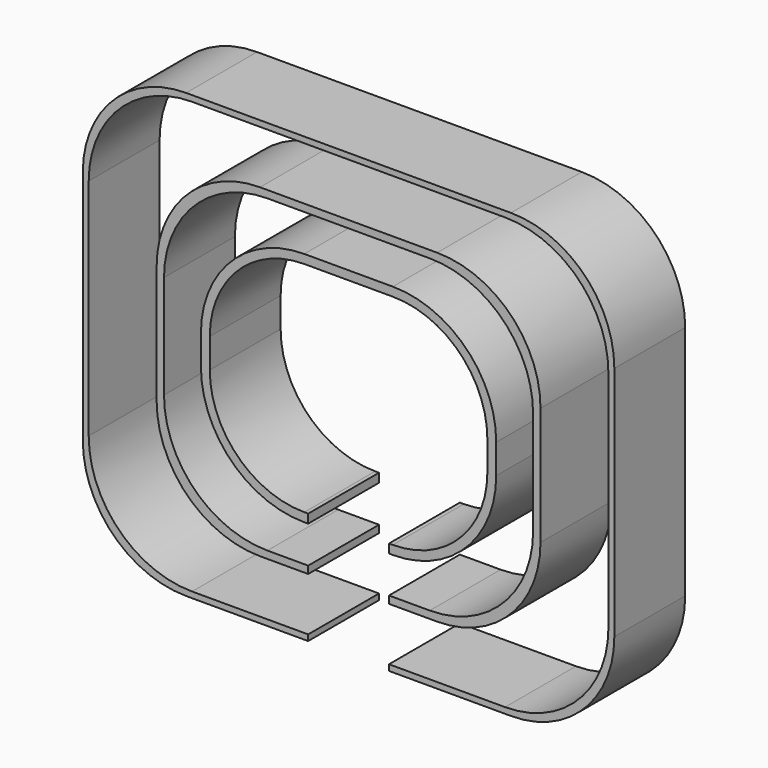
from build123d import *

# Parameters (mm, degrees)
F0_W      = 180
F0_H      = 150
F1_DEPTH  = 30
F2_T      = -2
F3_W      = 130
F3_H      = 110
F4_DEPTH  = 30
F5_T      = -2.5
F6_W      = 100
F6_H      = 80
F7_DEPTH  = 30
F8_R      = 35
F8_2_R    = 35
F8_3_R    = 35
F9_T      = -3
F10_W     = 27.3726535961
F10_H     = 91.242223978
F11_DEPTH = 30.001


with BuildPart() as f1:
    # F0 (on Front) → F1 (new body)
    with BuildSketch(Plane.XZ):
        Rectangle(F0_W, F0_H)
    extrude(amount=F1_DEPTH)

    # F2
    f2_openings = [f1.faces().sort_by_distance(p)[0] for p in [
        (0, -30, 0),
        (0, 0, 0),
    ]]
    offset(amount=F2_T, openings=f2_openings)

    # F8
    f8_edges = [f1.edges().sort_by_distance(p)[0] for p in [
        (-88, -15, 73),
        (-90, -15, 75),
        (90, -15, 75),
        (88, -15, 73),
        (88, -15, -73),
        (90, -15, -75),
        (-88, -15, -73),
        (-90, -15, -75),
    ]]
    fillet(f8_edges, radius=F8_R)


with BuildPart() as f4:
    # F3 (on face) → F4 (new body)
    with BuildSketch(Plane.XZ):
        Rectangle(F3_W, F3_H)
    extrude(amount=F4_DEPTH)

    # F5
    f5_openings = [f4.faces().sort_by_distance(p)[0] for p in [
        (0, -30, 0),
        (0, 0, 0),
    ]]
    offset(amount=F5_T, openings=f5_openings)

    # F8#2
    f8_2_edges = [f4.edges().sort_by_distance(p)[0] for p in [
        (-62.5, -15, 52.5),
        (-65, -15, 55),
        (-62.5, -15, -52.5),
        (-65, -15, -55),
        (62.5, -15, -52.5),
        (62.5, -15, 52.5),
        (65, -15, -55),
        (65, -15, 55),
    ]]
    fillet(f8_2_edges, radius=F8_2_R)


with BuildPart() as f7:
    # F6 (on face) → F7 (new body)
    with BuildSketch(Plane.XZ):
        Rectangle(F6_W, F6_H)
    extrude(amount=F7_DEPTH)

    # F8#3
    f8_3_edges = [f7.edges().sort_by_distance(p)[0] for p in [
        (50, -15, 40),
        (-50, -15, 40),
        (-50, -15, -40),
        (50, -15, -40),
    ]]
    fillet(f8_3_edges, radius=F8_3_R)

    # F9
    f9_openings = [f7.faces().sort_by_distance(p)[0] for p in [
        (0, -30, 0),
        (0, 0, 0),
    ]]
    offset(amount=F9_T, openings=f9_openings)


with BuildPart() as f11_tool:
    # F10 (on face) → F11 (new body, through all)
    with BuildSketch(Plane.XZ):
        with Locations((1.72295e-05, -79.0765881538)):
            Rectangle(F10_W, F10_H)
    extrude(amount=F11_DEPTH)


with BuildPart() as f1_1:
    add(f1.part)

    # F11: cut by f11_tool
    add(f11_tool.part, mode=Mode.SUBTRACT)


with BuildPart() as f4_1:
    add(f4.part)

    # F11: cut by f11_tool
    add(f11_tool.part, mode=Mode.SUBTRACT)


with BuildPart() as f7_1:
    add(f7.part)

    # F11: cut by f11_tool
    add(f11_tool.part, mode=Mode.SUBTRACT)


solid = Compound([f1_1.part, f4_1.part, f7_1.part])
